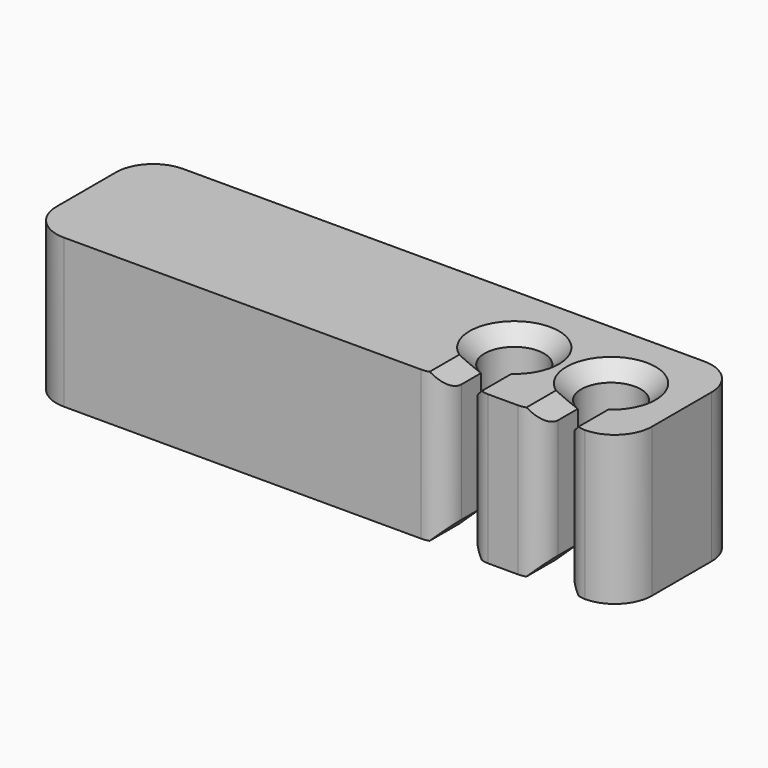
from build123d import *

# Parameters (mm, degrees)
F0_W     = 80
F0_H     = 20
F1_DEPTH = 20
F3_DEPTH = 20.001
F4_R     = 4
F5_DEPTH = 20.001
F6_SIZE  = 2
F7_R     = 3
F8_R     = 4.99999


# Not quite as in the source:
# - a fillet or chamfer is up to 0.001 mm smaller than in the source, because OpenCascade refuses the exact size


with BuildPart() as f1:
    # F0 (on Top) → F1 (new body)
    with BuildSketch(Plane.XY):
        Rectangle(F0_W, F0_H)
    extrude(amount=F1_DEPTH)

    # F2 (on face) → F3 (cut, through all)
    with BuildSketch(Plane.XY.offset(20)):
        with BuildLine():
            Line((29, -10), (32, -10))
            Line((32, -10), (32, 0))
            ThreePointArc((32, 0), (30.5, 1.5), (29, 0))
            Line((29, 0), (29, -10))
        make_face()
        with BuildLine():
            Line((16, -10), (19, -10))
            Line((19, -10), (19, 0))
            ThreePointArc((19, 0), (17.5, 1.5), (16, 0))
            Line((16, 0), (16, -10))
        make_face()
    extrude(amount=-F3_DEPTH, mode=Mode.SUBTRACT)

    # F4 (on face) → F5 (cut, through all)
    with BuildSketch(Plane.XY.offset(20)):
        with Locations((17.5, 0)):
            Circle(F4_R)
        with Locations((30.5, 0)):
            Circle(F4_R)
    extrude(amount=-F5_DEPTH, mode=Mode.SUBTRACT)

    # F6
    f6_edges = [f1.edges().sort_by_distance(p)[0] for p in [
        (17.5, 4, 20),
        (30.5, 4, 20),
        (17.5, 4, 0),
        (30.5, 4, 0),
        (16, -6.85405, 20),
        (19, -6.85405, 20),
        (29, -6.85405, 20),
        (32, -6.85405, 20),
        (16, -6.85405, 0),
        (19, -6.85405, 0),
        (29, -6.85405, 0),
        (32, -6.85405, 0),
    ]]
    chamfer(f6_edges, length=F6_SIZE)

    # F7
    f7_edges = [f1.edges().sort_by_distance(p)[0] for p in [
        (19, -10, 10),
        (29, -10, 10),
        (32, -10, 10),
        (16, -10, 10),
    ]]
    fillet(f7_edges, radius=F7_R)

    # F8 (radius 5 in the source; OpenCascade refuses exactly that, so slightly less here)
    f8_edges = [f1.edges().sort_by_distance(p)[0] for p in [
        (40, -10, 10),
        (40, 10, 10),
        (-40, 10, 10),
        (-40, -10, 10),
    ]]
    fillet(f8_edges, radius=F8_R)


solid = f1.part
